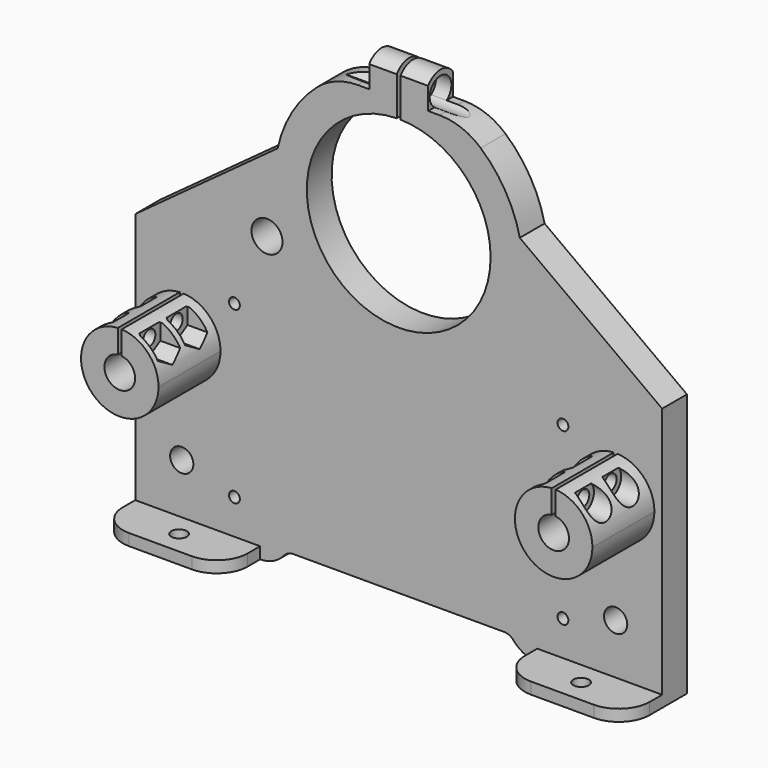
from build123d import *
from build123d import SkipClean  # not in build123d's __all__

# Parameters (mm, degrees)
F0_R           = 4.7625
F0_R_2         = 6.2865
F0_R_3         = 37.6555
F1_DEPTH       = 12.7
F2_R           = 63.5
F3_DEPTH       = 25.4
F4_R           = 12.7
F5_R           = 15.875
F5_R_2         = 6.2865
F6_DEPTH       = 31.75
F8_DEPTH       = 31.75
F9_R           = 3.175
F10_DEPTH      = 224.536
F12_DEPTH      = 83.185
F12_DEPTH_BACK = 83.185
F13_R          = 5.55625
F14_DEPTH      = 13.335
F15_R          = 5.55625
F16_DEPTH      = 13.335
F17_W          = 51.1538733715
F17_H          = 19.05
F17_R          = 3.175
F18_DEPTH      = 4.7498
F19_R          = 12.7
F20_R          = 50.8
F20_R_2        = 37.6555
F21_DEPTH      = 12.7
F22_W          = 1.5875
F22_H          = 25.6619900465
F23_DEPTH      = 25.4
F24_W          = 25.4
F24_H          = 9.9264993731
F25_DEPTH      = 25.4
F26_W          = 6.19125
F26_H          = 15.875
F27_DEPTH      = 12.7
F29_DEPTH      = 25.4
F29_DEPTH_BACK = 25.4
F31_DEPTH      = 6.19125
F33_DEPTH      = 6.19125
F34_R          = 25.4
F35_R          = 5.55625
F36_DEPTH      = 28.9306
F38_DEPTH      = 22.225
F39_R          = 2.2225
F40_DEPTH      = 25.4
F41_R          = 6.35
F42_DEPTH      = 25.4
F43_DEPTH      = 1.27
F44_DEPTH      = 1.27
F46_DEPTH      = 6.35
F48_DEPTH      = 6.35
F49_W          = 100.0235989526
F49_H          = 22.1718842693
F50_DEPTH      = 12.7
F51_R          = 5.08


# Not quite as in the source:
# - after a boolean that leaves OpenCascade's solid faulty, fix() repairs it


with BuildPart() as f1:
    # F0 (on Front) → F1 (new body)
    with BuildSketch(Plane.XZ):
        with BuildLine():
            Line((-107.95, 38.1), (-107.95, -69.85))
            Line((-107.95, -69.85), (107.95, -69.85))
            Line((107.95, -69.85), (107.95, 38.1))
            Line((107.95, 38.1), (22.4919418666, 100.6026023463))
            ThreePointArc((22.4919418666, 100.6026023463), (0, 107.95), (-22.4919418666, 100.6026023463))
            Line((-22.4919418666, 100.6026023463), (-107.95, 38.1))
        make_face()
        with Locations((-88.9, -44.45)):
            Circle(F0_R, mode=Mode.SUBTRACT)
        with Locations((-88.9, 0)):
            Circle(F0_R_2, mode=Mode.SUBTRACT)
        with Locations((88.9, -44.45)):
            Circle(F0_R, mode=Mode.SUBTRACT)
        with Locations((88.9, 0)):
            Circle(F0_R_2, mode=Mode.SUBTRACT)
        with Locations((0, 69.85)):
            Circle(F0_R_3, mode=Mode.SUBTRACT)
    extrude(amount=F1_DEPTH)

    # F2 (on face) → F3 (cut)
    with BuildSketch(Plane.XZ.offset(12.7)):
        with Locations((0, -107.95)):
            Circle(F2_R)
    extrude(amount=-F3_DEPTH, mode=Mode.SUBTRACT)

    # F4
    f4_edges = [f1.edges().sort_by_distance(p)[0] for p in [
        (-50.8, -6.35, -69.85),
        (50.8, -6.35, -69.85),
    ]]
    fillet(f4_edges, radius=F4_R)

    # F5 (on face) → F6 (join)
    with BuildSketch(Plane.XZ.offset(12.7)):
        with Locations((-88.9, 0)):
            Circle(F5_R)
        with Locations((-88.9, 0)):
            Circle(F5_R_2, mode=Mode.SUBTRACT)
        with Locations((88.9, 0)):
            Circle(F5_R)
        with Locations((88.9, 0)):
            Circle(F5_R_2, mode=Mode.SUBTRACT)
    extrude(amount=F6_DEPTH)

    # F7 (on face) → F8 (cut, through all)
    with BuildSketch(Plane.XZ.offset(44.45)):
        Polygon((-89.69375, 19.6568928659), (-89.69375, 1.7181718722), (-88.9, 1.7181718722), (-88.10625, 1.7181718722), (-88.10625, 19.6568928659), align=None)
        Polygon((89.69375, 20.8262372762), (88.10625, 20.8262372762), (88.10625, 3.0810327735), (88.9, 3.0810327735), (89.69375, 3.0810327735), align=None)
    extrude(amount=-F8_DEPTH, mode=Mode.SUBTRACT)

    # F9 (on face) → F10 (cut)
    with BuildSketch(Plane(origin=(-107.95, 0, 0), x_dir=(0, -1, 0), z_dir=(-1, 0, 0))):
        with Locations((36.5252, 11.1053438321)):
            Circle(F9_R)
        with Locations((22.5552, 11.1053438321)):
            Circle(F9_R)
    extrude(amount=-F10_DEPTH, mode=Mode.SUBTRACT)

    # F11 (on Right) → F12 (cut, two sides)
    with BuildSketch(Plane.YZ) as f12_sk:
        Polygon((-30.8059682334, 14.4073438321), (-36.5252, 17.7093438321), (-42.2444317666, 14.4073438321), (-42.2444317666, 7.8033438321), (-36.5252, 4.5013438321), (-30.8059682334, 7.8033438321), align=None)
        Polygon((-22.5552, 17.7093438321), (-28.2744317666, 14.4073438321), (-28.2744317666, 7.8033438321), (-22.5552, 4.5013438321), (-16.8359682334, 7.8033438321), (-16.8359682334, 14.4073438321), align=None)
    extrude(amount=-F12_DEPTH, mode=Mode.SUBTRACT)
    extrude(f12_sk.sketch, amount=F12_DEPTH_BACK, mode=Mode.SUBTRACT)

    # F13 (on face) → F14 (cut)
    with BuildSketch(Plane(origin=(-107.95, 0, 0), x_dir=(0, -1, 0), z_dir=(-1, 0, 0))):
        with Locations((22.5552, 11.1053438321)):
            Circle(F13_R)
        with Locations((36.5252, 11.1053438321)):
            Circle(F13_R)
    extrude(amount=-F14_DEPTH, mode=Mode.SUBTRACT)

    # F15 (on face) → F16 (cut)
    with BuildSketch(Plane.YZ.offset(107.95)):
        with Locations((-36.5252, 11.1053438321)):
            Circle(F15_R)
        with Locations((-22.5552, 11.1053438321)):
            Circle(F15_R)
    extrude(amount=-F16_DEPTH, mode=Mode.SUBTRACT)

    # F17 (on face) → F18 (join)
    with BuildSketch(Plane(origin=(0, 0, -69.85), x_dir=(1, 0, 0), z_dir=(0, 0, -1))):
        with Locations((82.3730633142, 22.225)):
            Rectangle(F17_W, F17_H)
        with Locations((82.3730633142, 22.225)):
            Circle(F17_R, mode=Mode.SUBTRACT)
        with Locations((-82.3730633142, 22.225)):
            Rectangle(F17_W, F17_H)
        with Locations((-82.3730633142, 22.225)):
            Circle(F17_R, mode=Mode.SUBTRACT)
    extrude(amount=-F18_DEPTH)

    # F19
    f19_edges = [f1.edges().sort_by_distance(p)[0] for p in [
        (56.796127, -31.75, -67.4751),
        (107.95, -31.75, -67.4751),
        (-56.796127, -31.75, -67.4751),
        (-107.95, -31.75, -67.4751),
    ]]
    fillet(f19_edges, radius=F19_R)

    # F20 (on face) → F21 (join)
    with BuildSketch(Plane.XZ.offset(12.7)):
        with Locations((0, 69.85)):
            Circle(F20_R)
        with Locations((0, 69.85)):
            Circle(F20_R_2, mode=Mode.SUBTRACT)
    extrude(amount=-F21_DEPTH)

    # F22 (on face) → F23 (cut)
    with BuildSketch(Plane.XZ.offset(12.7)):
        with Locations((0, 110.4765236378)):
            Rectangle(F22_W, F22_H)
    extrude(amount=-F23_DEPTH, mode=Mode.SUBTRACT)

    # F24 (on face) → F25 (cut)
    with BuildSketch(Plane.XZ.offset(12.7)):
        with Locations((-19.685, 119.2632496866)):
            Rectangle(F24_W, F24_H)
        with Locations((19.685, 119.2632496866)):
            Rectangle(F24_W, F24_H)
    extrude(amount=-F25_DEPTH, mode=Mode.SUBTRACT)

    # F26 (on face) → F27 (join)
    with BuildSketch(Plane.XZ.offset(12.7)):
        with Locations((-3.889375, 115.43463324)):
            Rectangle(F26_W, F26_H)
        with Locations((3.889375, 115.43463324)):
            Rectangle(F26_W, F26_H)
    extrude(amount=-F27_DEPTH)

    # F28 (on face) → F29 (cut, two sides)
    with BuildSketch(Plane.YZ.offset(-0.79375)) as f29_sk:
        with BuildLine():
            ThreePointArc((-6.35, 115.75213324), (-4.1049359697, 116.6820692097), (-3.175, 118.92713324))
            ThreePointArc((-3.175, 118.92713324), (-8.5950640303, 121.1721972702), (-6.35, 115.75213324))
        make_face()
    extrude(amount=-F29_DEPTH, mode=Mode.SUBTRACT)
    extrude(f29_sk.sketch, amount=F29_DEPTH_BACK, mode=Mode.SUBTRACT)

    # F30 (on face) → F31 (join, through all)
    with BuildSketch(Plane.YZ.offset(6.985)):
        with BuildLine():
            Line((-12.7, 123.37213324), (0, 123.37213324))
            ThreePointArc((0, 123.37213324), (-6.35, 126.678296056), (-12.7, 123.37213324))
        make_face()
    extrude(amount=-F31_DEPTH)

    # F32 (on face) → F33 (join, through all)
    with BuildSketch(Plane(origin=(-6.985, 0, 0), x_dir=(0, -1, 0), z_dir=(-1, 0, 0))):
        with BuildLine():
            Line((0, 123.37213324), (12.7, 123.37213324))
            ThreePointArc((12.7, 123.37213324), (6.35, 126.678296056), (0, 123.37213324))
        make_face()
    extrude(amount=-F33_DEPTH)

    # F34
    f34_edges = [f1.edges().sort_by_distance(p)[0] for p in [
        (-24.593444, -6.35, 114.3),
        (24.593444, -6.35, 114.3),
    ]]
    fillet(f34_edges, radius=F34_R)

    # F35 (on face) → F36 (cut)
    with BuildSketch(Plane.YZ.offset(6.985)):
        with Locations((-6.35, 118.92713324)):
            Circle(F35_R)
    extrude(amount=F36_DEPTH, mode=Mode.SUBTRACT)

    # F37 (on face) → F38 (cut)
    with BuildSketch(Plane(origin=(-6.985, 0, 0), x_dir=(0, -1, 0), z_dir=(-1, 0, 0))):
        Polygon((6.35, 125.53113324), (0.6307682334, 122.22913324), (0.6307682334, 115.62513324), (6.35, 112.32313324), (12.0692317666, 115.62513324), (12.0692317666, 122.22913324), align=None)
    extrude(amount=F38_DEPTH, mode=Mode.SUBTRACT)

    # F39 (on face) → F40 (cut)
    with BuildSketch(Plane.XZ.offset(12.7)):
        with Locations((-67.31, -50.8)):
            Circle(F39_R)
        with Locations((-67.31, 19.05)):
            Circle(F39_R)
        with Locations((67.31, 19.05)):
            Circle(F39_R)
        with Locations((67.31, -50.8)):
            Circle(F39_R)
    extrude(amount=-F40_DEPTH, mode=Mode.SUBTRACT)

    # F41 (on face) → F42 (cut)
    with BuildSketch(Plane.XZ.offset(12.7)):
        with Locations((-53.975, 47.625)):
            Circle(F41_R)
    extrude(amount=-F42_DEPTH, mode=Mode.SUBTRACT)

    # F43 (cut): a face of the model
    f43_faces = [f1.faces().sort_by_distance(p)[0] for p in [
        (6.985, -11.0629817979, 114.4839503291),
    ]]
    extrude(f43_faces, amount=-F43_DEPTH, mode=Mode.SUBTRACT)

    # F44 (cut): a face of the model
    f44_faces = [f1.faces().sort_by_distance(p)[0] for p in [
        (-6.985, -12.5083334407, 118.83606662),
    ]]
    extrude(f44_faces, amount=-F44_DEPTH, mode=Mode.SUBTRACT)

    # F45 (on face) → F46 (join)
    with BuildSketch(Plane.YZ.offset(5.715)):
        with BuildLine():
            Line((-3.2740364043, 114.3), (0, 114.3))
            Line((0, 114.3), (0, 123.37213324))
            ThreePointArc((0, 123.37213324), (-6.35, 126.678296056), (-12.7, 123.37213324))
            Line((-12.7, 123.37213324), (-12.7, 114.3))
            Line((-12.7, 114.3), (-9.4259635957, 114.3))
            ThreePointArc((-9.4259635957, 114.3), (-6.35, 124.48338324), (-3.2740364043, 114.3))
        make_face()
    with SkipClean():  # cleaning this boolean's faces spoils the solid; the shape is the same uncleaned
        extrude(amount=F46_DEPTH)

    # F47 (on face) → F48 (join)
    with BuildSketch(Plane(origin=(-5.715, 0, 0), x_dir=(0, -1, 0), z_dir=(-1, 0, 0))):
        with BuildLine():
            Line((0, 114.3), (2.9259663318, 114.3))
            Line((2.9259663318, 114.3), (0.6307682334, 115.62513324))
            Line((0.6307682334, 115.62513324), (0.6307682334, 122.22913324))
            Line((0.6307682334, 122.22913324), (6.35, 125.53113324))
            Line((6.35, 125.53113324), (12.0692317666, 122.22913324))
            Line((12.0692317666, 122.22913324), (12.0692317666, 115.62513324))
            Line((12.0692317666, 115.62513324), (9.7740336682, 114.3))
            Line((9.7740336682, 114.3), (12.7, 114.3))
            Line((12.7, 114.3), (12.7, 123.37213324))
            ThreePointArc((12.7, 123.37213324), (6.35, 126.678296056), (0, 123.37213324))
            Line((0, 123.37213324), (0, 114.3))
        make_face()
    extrude(amount=F48_DEPTH)

    add(f1.part.fix(), mode=Mode.REPLACE)

    # F49 (on face) → F50 (join)
    with BuildSketch(Plane.XZ.offset(12.7)):
        with Locations((0, -52.4140578653)):
            Rectangle(F49_W, F49_H)
    extrude(amount=-F50_DEPTH)

    # F51
    f51_edges = [f1.edges().sort_by_distance(p)[0] for p in [
        (45.348071, -6.35, -63.5),
        (-45.348071, -6.35, -63.5),
    ]]
    fillet(f51_edges, radius=F51_R)


solid = f1.part
